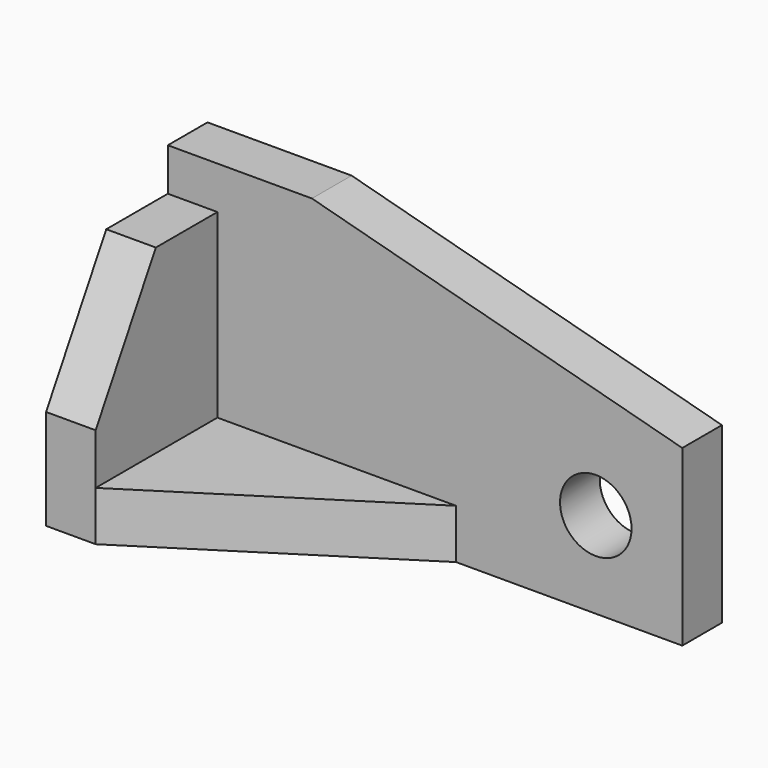
from build123d import *

# Parameters (mm, degrees)
F0_R     = 7.874
F0_W     = 10.922
F0_H     = 22.098
F0_H_2   = 28.702
F1_DEPTH = 10.922
F2_DEPTH = 33.528
F4_DEPTH = 25.4
F3_W     = 33.528
F3_H     = 10.922
F5_DEPTH = 52.578
F7_DEPTH = 25.4


with BuildPart() as f1:
    # F0 (on Front) → F1 (new body)
    with BuildSketch(Plane.XZ):
        Polygon((-7.7014979906, 38.1), (-39.4514979906, 38.1), (-39.4514979906, 28.702), (-28.5294979906, 28.702), (-28.5294979906, 0), (-28.5294979906, -22.098), (-7.7014979906, -22.098), align=None)
        Polygon((73.8835578219, 16.2393501806), (-7.7014979906, 38.1), (-7.7014979906, -22.098), (73.8835578219, -22.098), align=None)
        with Locations((54.8335578219, -3.048)):
            Circle(F0_R, mode=Mode.SUBTRACT)
        with Locations((-33.9904979906, -11.049)):
            Rectangle(F0_W, F0_H)
        with Locations((-33.9904979906, 14.351)):
            Rectangle(F0_W, F0_H_2)
    extrude(amount=-F1_DEPTH)

    # F0 (on Front) → F2 (join)
    with BuildSketch(Plane.XZ):
        with Locations((-33.9904979906, 14.351)):
            Rectangle(F0_W, F0_H_2)
        with Locations((-33.9904979906, -11.049)):
            Rectangle(F0_W, F0_H)
    extrude(amount=F2_DEPTH)

    # F3 (on face) → F4 (cut)
    with BuildSketch(Plane.YZ.offset(-28.5294979906)):
        Polygon((-33.528, 28.702), (-33.528, 0), (-16.9568925737, 28.702), align=None)
    extrude(amount=-F4_DEPTH, mode=Mode.SUBTRACT)

    # F3 (on face) → F5 (join)
    with BuildSketch(Plane.YZ.offset(-28.5294979906)):
        with Locations((-16.764, -16.637)):
            Rectangle(F3_W, F3_H)
    extrude(amount=F5_DEPTH)

    # F6 (on face) → F7 (cut)
    with BuildSketch(Plane.XY.offset(-11.176)):
        Polygon((24.0485020094, 0), (-28.5294979906, -33.528), (24.0485020094, -33.528), align=None)
    extrude(amount=-F7_DEPTH, mode=Mode.SUBTRACT)


solid = f1.part
